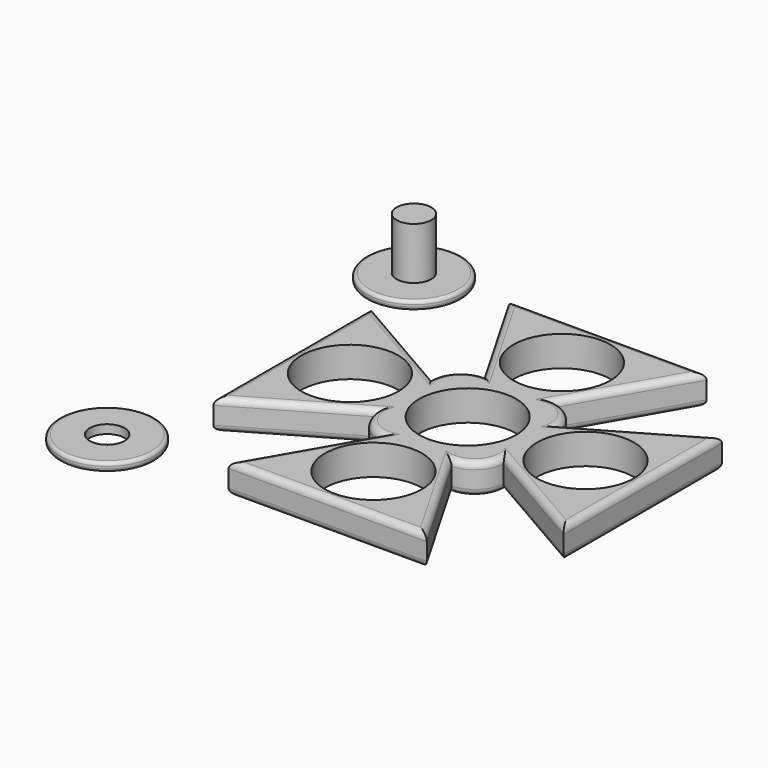
from build123d import *

# Parameters (mm, degrees)
F0_R      = 11.2
F1_DEPTH  = 7
F2_R      = 1.499
F3_R      = 1.5
F4_R      = 11
F5_DEPTH  = 2
F6_R      = 4.0005
F7_DEPTH  = 12
F8_R      = 0.762
F9_R      = 11
F10_DEPTH = 2
F11_R     = 4.013
F12_DEPTH = 2
F13_R     = 4.013
F14_DEPTH = 2
F15_R     = 0.762


# Not quite as in the source:
# - a fillet or chamfer is up to 0.001 mm smaller than in the source, because OpenCascade refuses the exact size


with BuildPart() as f1:
    # F0 (on Top) → F1 (new body)
    with BuildSketch(Plane.XY):
        with BuildLine():
            Line((-40.3780304611, 22.8630706599), (-40.3780304611, -22.8630706599))
            Line((-40.3780304611, -22.8630706599), (-14.6492169979, -8.008533281))
            ThreePointArc((-14.6492169979, -8.008533281), (-12.6082129963, -12.5990680914), (-8.0748202901, -14.7640294654))
            Line((-8.0748202901, -14.7640294654), (-22.8630706599, -40.3780304611))
            Line((-22.8630706599, -40.3780304611), (22.8630706599, -40.3780304611))
            Line((22.8630706599, -40.3780304611), (8.008533281, -14.6492169979))
            ThreePointArc((8.008533281, -14.6492169979), (12.5990680914, -12.6082129963), (14.7640294654, -8.0748202901))
            Line((14.7640294654, -8.0748202901), (40.3780304611, -22.8630706599))
            Line((40.3780304611, -22.8630706599), (40.3780304611, 22.8630706599))
            Line((40.3780304611, 22.8630706599), (14.6492169979, 8.008533281))
            ThreePointArc((14.6492169979, 8.008533281), (12.6082129963, 12.5990680914), (8.0748202901, 14.7640294654))
            Line((8.0748202901, 14.7640294654), (22.8630706599, 40.3780304611))
            Line((22.8630706599, 40.3780304611), (-22.8630706599, 40.3780304611))
            Line((-22.8630706599, 40.3780304611), (-8.008533281, 14.6492169979))
            ThreePointArc((-8.008533281, 14.6492169979), (-12.5990680914, 12.6082129963), (-14.7640294654, 8.0748202901))
            Line((-14.7640294654, 8.0748202901), (-40.3780304611, 22.8630706599))
        make_face()
        with Locations((0, -27.1780304611)):
            Circle(F0_R, mode=Mode.SUBTRACT)
        with Locations((-27.1780304611, 0)):
            Circle(F0_R, mode=Mode.SUBTRACT)
        Circle(F0_R, mode=Mode.SUBTRACT)
        with Locations((27.1780304611, 0)):
            Circle(F0_R, mode=Mode.SUBTRACT)
        with Locations((0, 27.1780304611)):
            Circle(F0_R, mode=Mode.SUBTRACT)
    extrude(amount=F1_DEPTH)

    # F2 (radius 1.5 in the source; OpenCascade refuses exactly that, so slightly less here)
    f2_edges = [f1.edges().sort_by_distance(p)[0] for p in [
        (0, -40.37803, 7),
        (-15.468945, -27.57103, 7),
        (-12.608213, -12.599068, 7),
        (-27.513624, -15.435802, 7),
        (-40.37803, 0, 7),
        (-27.57103, 15.468945, 7),
        (-12.599068, 12.608213, 7),
        (-15.435802, 27.513624, 7),
        (0, 40.37803, 7),
        (15.468945, 27.57103, 7),
        (27.513624, 15.435802, 7),
        (12.608213, 12.599068, 7),
        (40.37803, 0, 7),
        (27.57103, -15.468945, 7),
        (12.599068, -12.608213, 7),
        (15.435802, -27.513624, 7),
    ]]
    fillet(f2_edges, radius=F2_R)

    # F3
    f3_edges = [f1.edges().sort_by_distance(p)[0] for p in [
        (0, -40.37803, 0),
        (15.435802, -27.513624, 0),
        (-15.468945, -27.57103, 0),
        (-40.37803, 0, 0),
        (-27.513624, -15.435802, 0),
        (-27.57103, 15.468945, 0),
        (-12.608213, -12.599068, 0),
        (-12.599068, 12.608213, 0),
        (-15.435802, 27.513624, 0),
        (0, 40.37803, 0),
        (15.468945, 27.57103, 0),
        (12.608213, 12.599068, 0),
        (27.513624, 15.435802, 0),
        (40.37803, 0, 0),
        (27.57103, -15.468945, 0),
        (12.599068, -12.608213, 0),
    ]]
    fillet(f3_edges, radius=F3_R)

    # F11 (on face) → F12 (cut)
    with BuildSketch(Plane.XY.offset(2)):
        with Locations((-52.4518378079, -38.4357832372)):
            Circle(F11_R)
    extrude(amount=F12_DEPTH, mode=Mode.SUBTRACT)


with BuildPart() as f5:
    # F4 (on Top) → F5 (new body)
    with BuildSketch(Plane.XY):
        with Locations((-48.6949570477, 45.3715622425)):
            Circle(F4_R)
    extrude(amount=F5_DEPTH)

    # F6 (on face) → F7 (join)
    with BuildSketch(Plane.XY.offset(2)):
        with Locations((-48.6949570477, 45.3715622425)):
            Circle(F6_R)
    extrude(amount=F7_DEPTH)

    # F8
    f8_edges = [f5.edges().sort_by_distance(p)[0] for p in [
        (-59.694957, 45.371562, 2),
        (-59.694957, 45.371562, 0),
    ]]
    fillet(f8_edges, radius=F8_R)


with BuildPart() as f10:
    # F9 (on Top) → F10 (new body)
    with BuildSketch(Plane.XY):
        with Locations((-52.4518378079, -38.4357832372)):
            Circle(F9_R)
    extrude(amount=F10_DEPTH)

    # F13 (on face) → F14 (cut)
    with BuildSketch(Plane.XY.offset(2)):
        with Locations((-52.4518378079, -38.4357832372)):
            Circle(F13_R)
    extrude(amount=-F14_DEPTH, mode=Mode.SUBTRACT)

    # F15
    f15_edges = [f10.edges().sort_by_distance(p)[0] for p in [
        (-63.451838, -38.435783, 2),
        (-63.451838, -38.435783, 0),
    ]]
    fillet(f15_edges, radius=F15_R)


solid = Compound([f1.part, f5.part, f10.part])
